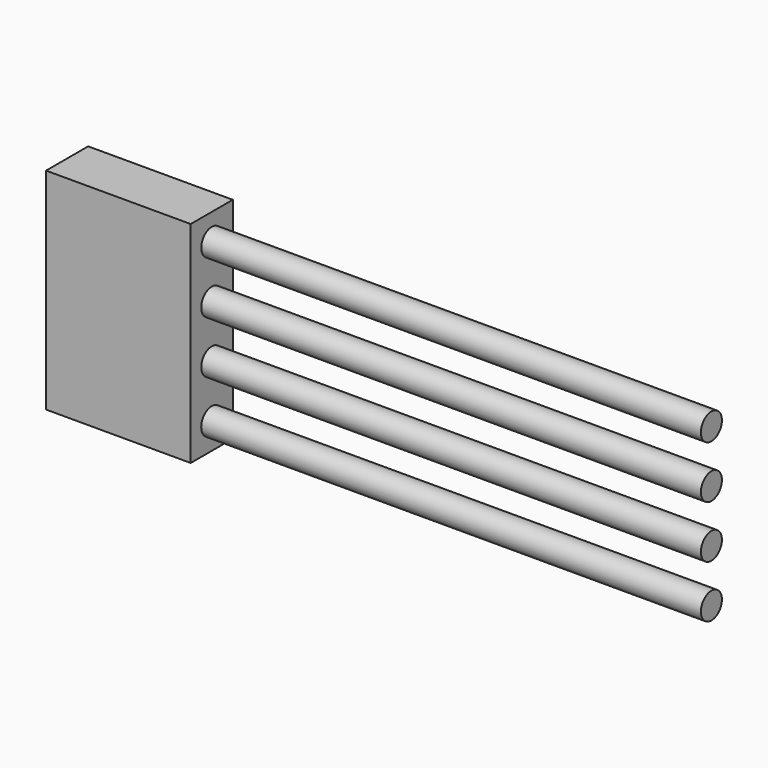
from build123d import *

# Parameters (mm, degrees)
F0_W      = 406.4
F0_H      = 12.7
F0_W_2    = 139.7
F0_H_2    = 38.1
F2_DEPTH  = 25.4
F3_DEPTH  = 25.4
F4_DEPTH  = 76.2
F5_W      = 76.2
F5_H      = 50.8
F6_DEPTH  = 139.7
F7_R      = 12.7
F8_DEPTH  = 482.6
F9_DEPTH  = 7.62
F10_W     = 56.2998503447
F10_H     = 25.4
F11_DEPTH = 2.54
F12_W     = 51.2198503447
F12_H     = 20.32
F13_DEPTH = 2.54
F14_DEPTH = 12.7
F15_DEPTH = 12.7
F18_DEPTH = 76.2
F20_DEPTH = 127
F19_W     = 0.508
F19_H     = 0.5186796188
F21_DEPTH = 101.6
F22_DEPTH = 2.54
F17_W     = 49.1785109043
F17_H     = 5.08
F23_DEPTH = 17.78
F24_R     = 2.54
F25_R     = 2.54


with BuildPart() as f1:
    # F0 (on Top) → F1 (revolve)
    with BuildSketch(Plane.XY):
        with Locations((63.891280989, 63.9939386676)):
            Rectangle(F0_W, F0_H)
    revolve(axis=Axis((63.891280989, 70.3439386676, 0), (-1, 0, 0)))

    # F0 (on Top) → F2 (join)
    with BuildSketch(Plane.XY):
        with Locations((-209.158719011, 89.3939386676)):
            Rectangle(F0_W_2, F0_H_2)
        Polygon((-139.308719011, 57.6439386676), (-139.308719011, 70.3439386676), (-279.008719011, 70.3439386676), (-279.008719011, 32.2439386676), (-139.308719011, 32.2439386676), align=None)
    extrude(amount=F2_DEPTH)

    # F0 (on Top) → F3 (join)
    with BuildSketch(Plane.XY):
        with Locations((-209.158719011, 89.3939386676)):
            Rectangle(F0_W_2, F0_H_2)
        Polygon((-139.308719011, 57.6439386676), (-139.308719011, 70.3439386676), (-279.008719011, 70.3439386676), (-279.008719011, 32.2439386676), (-139.308719011, 32.2439386676), align=None)
    extrude(amount=-F3_DEPTH)

    # F4 (add): a face of the model
    f4_faces = [f1.faces().sort_by_distance(p)[0] for p in [
        (267.091280989, 70.3439386676, 0),
    ]]
    extrude(f4_faces, amount=F4_DEPTH)

    # F5 (on face) → F6 (join)
    with BuildSketch(Plane.YZ.offset(-139.308719011)):
        with Locations((70.3439386676, 152.4)):
            Rectangle(F5_W, F5_H)
        with Locations((70.3439386676, 101.6)):
            Rectangle(F5_W, F5_H)
        with Locations((70.3439386676, 50.8)):
            Rectangle(F5_W, F5_H)
    extrude(amount=-F6_DEPTH)

    # F7 (on face) → F8 (join)
    with BuildSketch(Plane.YZ.offset(-139.308719011)):
        with Locations((70.3439386676, 50.8)):
            Circle(F7_R)
        with Locations((70.3439386676, 101.6)):
            Circle(F7_R)
        with Locations((70.3439386676, 152.4)):
            Circle(F7_R)
    extrude(amount=F8_DEPTH)

    # F9 (add): faces of the model
    f9_faces = [f1.faces().sort_by_distance(p)[0] for p in [
        (-209.158719011, 108.4439386676, 0),
        (-209.158719011, 108.4439386676, 101.6),
    ]]
    extrude(f9_faces, amount=-F9_DEPTH)

    # F10 (on face) → F11 (join)
    with BuildSketch(Plane(origin=(0, 0, -25.4), x_dir=(1, 0, 0), z_dir=(0, 0, -1))):
        with Locations((-236.669190228, -70.3439386676)):
            Rectangle(F10_W, F10_H)
    extrude(amount=F11_DEPTH)

    # F12 (on face) → F13 (cut)
    with BuildSketch(Plane(origin=(0, 0, -27.94), x_dir=(1, 0, 0), z_dir=(0, 0, -1))):
        with Locations((-236.669190228, -70.3439386676)):
            Rectangle(F12_W, F12_H)
    extrude(amount=-F13_DEPTH, mode=Mode.SUBTRACT)

    # F14 (cut): faces of the model
    f14_faces = [f1.faces().sort_by_distance(p)[0] for p in [
        (-209.158719011, 108.4439386676, 0),
        (-209.158719011, 108.4439386676, 101.6),
    ]]
    extrude(f14_faces, amount=-F14_DEPTH, mode=Mode.SUBTRACT)

    # F15 (cut): faces of the model
    f15_faces = [f1.faces().sort_by_distance(p)[0] for p in [
        (-209.158719011, 32.2439386676, 0),
        (-209.158719011, 32.2439386676, 101.6),
    ]]
    extrude(f15_faces, amount=-F15_DEPTH, mode=Mode.SUBTRACT)

    # F17 (on face) → F23 (join)
    with BuildSketch(Plane(origin=(0, 95.7439386676, 0), x_dir=(-1, 0, 0), z_dir=(0, 1, 0))):
        with Locations((192.8136348724, 124.46)):
            Rectangle(F17_W, F17_H)
        with Locations((192.8136348724, 129.54)):
            Rectangle(F17_W, F17_H)
    extrude(amount=F23_DEPTH)

    # F24
    f24_edges = [f1.edges().sort_by_distance(p)[0] for p in [
        (-192.813635, 113.523939, 121.92),
    ]]
    fillet(f24_edges, radius=F24_R)

    # F25
    f25_edges = [f1.edges().sort_by_distance(p)[0] for p in [
        (-192.813635, 113.523939, 132.08),
    ]]
    fillet(f25_edges, radius=F25_R)


with BuildPart() as f18:
    # F16 (on face) → F18 (new body)
    with BuildSketch(Plane.YZ.offset(-139.308719011)):
        with BuildLine():
            ThreePointArc((125.0336358821, 25.4), (124.4865948415, 27.9784040248), (122.9397249166, 30.1125583423))
            Line((122.9397249166, 30.1125583423), (118.6836358821, 25.4))
            Line((118.6836358821, 25.4), (122.9397249166, 20.6874416577))
            ThreePointArc((122.9397249166, 20.6874416577), (124.4865948415, 22.8215959752), (125.0336358821, 25.4))
        make_face()
        with BuildLine():
            Line((122.9397249166, 20.6874416577), (118.6836358821, 25.4))
            Line((118.6836358821, 25.4), (114.4275468475, 20.6874416577))
            ThreePointArc((114.4275468475, 20.6874416577), (118.6836358821, 19.05), (122.9397249166, 20.6874416577))
        make_face()
        with BuildLine():
            Line((118.6836358821, 25.4), (114.4275468475, 30.1125583423))
            ThreePointArc((114.4275468475, 30.1125583423), (112.3336358821, 25.4), (114.4275468475, 20.6874416577))
            Line((114.4275468475, 20.6874416577), (118.6836358821, 25.4))
        make_face()
        with BuildLine():
            ThreePointArc((122.9397249166, 30.1125583423), (118.6836358821, 31.75), (114.4275468475, 30.1125583423))
            Line((114.4275468475, 30.1125583423), (118.6836358821, 25.4))
            Line((118.6836358821, 25.4), (122.9397249166, 30.1125583423))
        make_face()
    extrude(amount=-F18_DEPTH)


with BuildPart() as f18b:
    # F16 (on face) → F18, piece 2 (new body)
    with BuildSketch(Plane.YZ.offset(-139.308719011)):
        with BuildLine():
            ThreePointArc((125.0336358821, 76.2), (124.4865948415, 78.7784040248), (122.9397249166, 80.9125583423))
            Line((122.9397249166, 80.9125583423), (118.6836358821, 76.2))
            Line((118.6836358821, 76.2), (122.9397249166, 71.4874416577))
            ThreePointArc((122.9397249166, 71.4874416577), (124.4865948415, 73.6215959752), (125.0336358821, 76.2))
        make_face()
        with BuildLine():
            Line((118.6836358821, 76.2), (114.4275468475, 71.4874416577))
            ThreePointArc((114.4275468475, 71.4874416577), (118.6836358821, 69.85), (122.9397249166, 71.4874416577))
            Line((122.9397249166, 71.4874416577), (118.6836358821, 76.2))
        make_face()
        with BuildLine():
            Line((118.6836358821, 76.2), (114.4275468475, 80.9125583423))
            ThreePointArc((114.4275468475, 80.9125583423), (112.3336358821, 76.2), (114.4275468475, 71.4874416577))
            Line((114.4275468475, 71.4874416577), (118.6836358821, 76.2))
        make_face()
        with BuildLine():
            ThreePointArc((122.9397249166, 80.9125583423), (118.6836358821, 82.55), (114.4275468475, 80.9125583423))
            Line((114.4275468475, 80.9125583423), (118.6836358821, 76.2))
            Line((118.6836358821, 76.2), (122.9397249166, 80.9125583423))
        make_face()
    extrude(amount=-F18_DEPTH)


with BuildPart() as f18c:
    # F16 (on face) → F18, piece 3 (new body)
    with BuildSketch(Plane.YZ.offset(-139.308719011)):
        with BuildLine():
            ThreePointArc((125.0336358821, 127), (124.4865948415, 129.5784040248), (122.9397249166, 131.7125583423))
            Line((122.9397249166, 131.7125583423), (118.6836358821, 127))
            Line((118.6836358821, 127), (122.9397249166, 122.2874416577))
            ThreePointArc((122.9397249166, 122.2874416577), (124.4865948415, 124.4215959752), (125.0336358821, 127))
        make_face()
        with BuildLine():
            Line((118.6836358821, 127), (114.4275468475, 122.2874416577))
            ThreePointArc((114.4275468475, 122.2874416577), (118.6836358821, 120.65), (122.9397249166, 122.2874416577))
            Line((122.9397249166, 122.2874416577), (118.6836358821, 127))
        make_face()
        with BuildLine():
            Line((118.6836358821, 127), (114.4275468475, 131.7125583423))
            ThreePointArc((114.4275468475, 131.7125583423), (112.3336358821, 127), (114.4275468475, 122.2874416577))
            Line((114.4275468475, 122.2874416577), (118.6836358821, 127))
        make_face()
        with BuildLine():
            ThreePointArc((122.9397249166, 131.7125583423), (118.6836358821, 133.35), (114.4275468475, 131.7125583423))
            Line((114.4275468475, 131.7125583423), (118.6836358821, 127))
            Line((118.6836358821, 127), (122.9397249166, 131.7125583423))
        make_face()
    extrude(amount=-F18_DEPTH)

    # F19 (on face) → F20 (cut)
    with BuildSketch(Plane.YZ.offset(-139.308719011)):
        with BuildLine():
            ThreePointArc((118.3923785006, 132.0716436328), (115.0812718007, 130.5818114168), (113.6104088057, 127.2622346878))
            Line((113.6104088057, 127.2622346878), (118.3923785006, 127.2622346878))
            Line((118.3923785006, 127.2622346878), (118.3923785006, 131.1406195164))
            Line((118.3923785006, 131.1406195164), (118.3923785006, 132.0716436328))
        make_face()
        with BuildLine():
            Line((118.3923785006, 126.743555069), (113.610112846, 126.743555069))
            ThreePointArc((113.610112846, 126.743555069), (115.0792285984, 123.4202446824), (118.3923785006, 121.9283563672))
            Line((118.3923785006, 121.9283563672), (118.3923785006, 126.743555069))
        make_face()
        with BuildLine():
            Line((123.7571589181, 126.743555069), (118.9003785006, 126.743555069))
            Line((118.9003785006, 126.743555069), (118.9003785006, 121.9246258623))
            ThreePointArc((118.9003785006, 121.9246258623), (122.2616587088, 123.3938729014), (123.7571589181, 126.743555069))
        make_face()
        with BuildLine():
            Line((118.9003785006, 131.1406195164), (118.9003785006, 127.2622346878))
            Line((118.9003785006, 127.2622346878), (123.7568629584, 127.2622346878))
            ThreePointArc((123.7568629584, 127.2622346878), (122.259600463, 130.6081681385), (118.9003785006, 132.0753741377))
            Line((118.9003785006, 132.0753741377), (118.9003785006, 131.1406195164))
        make_face()
    extrude(amount=-F20_DEPTH, mode=Mode.SUBTRACT)

    # F19 (on face) → F21 (cut)
    with BuildSketch(Plane.YZ.offset(-139.308719011)):
        with BuildLine():
            Line((118.9003785006, 126.743555069), (118.3923785006, 126.743555069))
            Line((118.3923785006, 126.743555069), (118.3923785006, 121.9283563672))
            ThreePointArc((118.3923785006, 121.9283563672), (118.6463318388, 121.9201369695), (118.9003785006, 121.9246258623))
            Line((118.9003785006, 121.9246258623), (118.9003785006, 126.743555069))
        make_face()
        with BuildLine():
            Line((118.3923785006, 127.2622346878), (113.6104088057, 127.2622346878))
            ThreePointArc((113.6104088057, 127.2622346878), (113.603636709, 127.0028986581), (113.610112846, 126.743555069))
            Line((113.610112846, 126.743555069), (118.3923785006, 126.743555069))
            Line((118.3923785006, 126.743555069), (118.3923785006, 127.2622346878))
        make_face()
        with BuildLine():
            Line((118.3923785006, 131.1406195164), (118.3923785006, 127.2622346878))
            Line((118.3923785006, 127.2622346878), (118.9003785006, 127.2622346878))
            Line((118.9003785006, 127.2622346878), (118.9003785006, 131.1406195164))
            Line((118.9003785006, 131.1406195164), (118.9003785006, 132.0753741377))
            ThreePointArc((118.9003785006, 132.0753741377), (118.6463318388, 132.0798630305), (118.3923785006, 132.0716436328))
            Line((118.3923785006, 132.0716436328), (118.3923785006, 131.1406195164))
        make_face()
        with BuildLine():
            Line((123.7568629584, 127.2622346878), (118.9003785006, 127.2622346878))
            Line((118.9003785006, 127.2622346878), (118.9003785006, 126.743555069))
            Line((118.9003785006, 126.743555069), (123.7571589181, 126.743555069))
            ThreePointArc((123.7571589181, 126.743555069), (123.7620163829, 126.8717366442), (123.7636358821, 127))
            ThreePointArc((123.7636358821, 127), (123.7619423689, 127.1311610689), (123.7568629584, 127.2622346878))
        make_face()
        with Locations((118.6463785006, 127.0028948784)):
            Rectangle(F19_W, F19_H)
    extrude(amount=-F21_DEPTH, mode=Mode.SUBTRACT)

    # F19 (on face) → F22 (join)
    with BuildSketch(Plane.YZ.offset(-139.308719011)):
        with BuildLine():
            Line((118.3923785006, 127.2622346878), (113.6104088057, 127.2622346878))
            ThreePointArc((113.6104088057, 127.2622346878), (113.603636709, 127.0028986581), (113.610112846, 126.743555069))
            Line((113.610112846, 126.743555069), (118.3923785006, 126.743555069))
            Line((118.3923785006, 126.743555069), (118.3923785006, 127.2622346878))
        make_face()
        with BuildLine():
            Line((118.3923785006, 131.1406195164), (118.3923785006, 127.2622346878))
            Line((118.3923785006, 127.2622346878), (118.9003785006, 127.2622346878))
            Line((118.9003785006, 127.2622346878), (118.9003785006, 131.1406195164))
            Line((118.9003785006, 131.1406195164), (118.9003785006, 132.0753741377))
            ThreePointArc((118.9003785006, 132.0753741377), (118.6463318388, 132.0798630305), (118.3923785006, 132.0716436328))
            Line((118.3923785006, 132.0716436328), (118.3923785006, 131.1406195164))
        make_face()
        with BuildLine():
            Line((118.9003785006, 126.743555069), (118.3923785006, 126.743555069))
            Line((118.3923785006, 126.743555069), (118.3923785006, 121.9283563672))
            ThreePointArc((118.3923785006, 121.9283563672), (118.6463318388, 121.9201369695), (118.9003785006, 121.9246258623))
            Line((118.9003785006, 121.9246258623), (118.9003785006, 126.743555069))
        make_face()
        with BuildLine():
            Line((123.7568629584, 127.2622346878), (118.9003785006, 127.2622346878))
            Line((118.9003785006, 127.2622346878), (118.9003785006, 126.743555069))
            Line((118.9003785006, 126.743555069), (123.7571589181, 126.743555069))
            ThreePointArc((123.7571589181, 126.743555069), (123.7620163829, 126.8717366442), (123.7636358821, 127))
            ThreePointArc((123.7636358821, 127), (123.7619423689, 127.1311610689), (123.7568629584, 127.2622346878))
        make_face()
        with Locations((118.6463785006, 127.0028948784)):
            Rectangle(F19_W, F19_H)
    extrude(amount=-F22_DEPTH)


solid = Compound([f1.part, f18.part, f18b.part, f18c.part])
